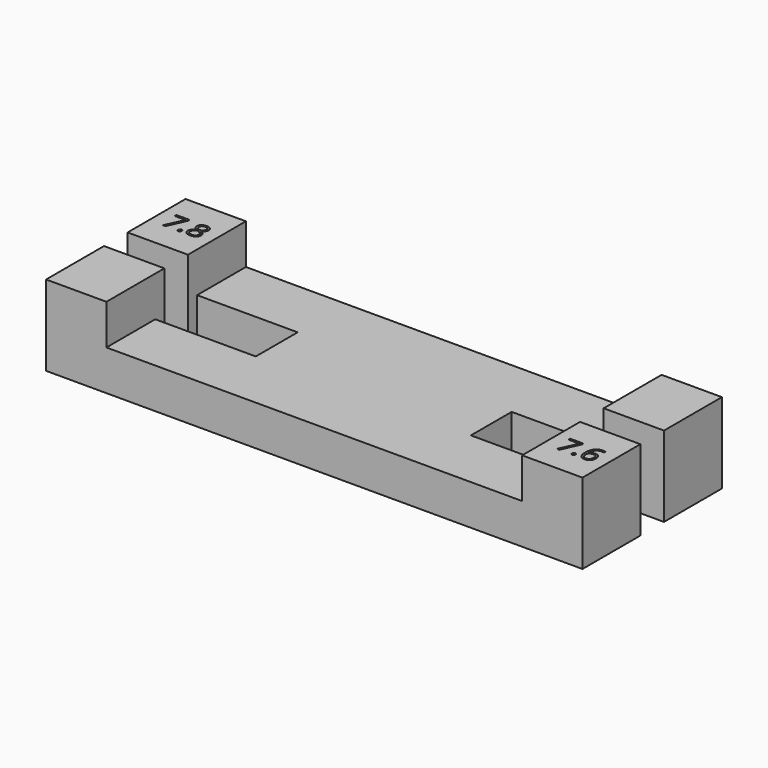
from build123d import *

# Parameters (mm, degrees)
F1_DEPTH     = 12
F2_W         = 62
F2_H         = 5
F3_DEPTH     = 6
F4_W         = 15
F4_H         = 1.7
F4_H_2       = 1.6
F5_DEPTH     = 25
F6_TEXT_SIZE = 4.1666666667
F7_DEPTH     = 5
F8_TEXT_SIZE = 4.1666666667
F9_DEPTH     = 5


# Not quite as in the source:
# - Text() gives the source's letters only with a copy of the font that has no kerning and outlines rounded to 1/6400 em; it was checked with that copy


with BuildPart() as f1:
    # F0 (on Top) → F1 (new body)
    with BuildSketch(Plane.XY):
        Polygon((40, 2.2), (40, 13), (-40, 13), (-40, 2.2), (-16, 2.2), (-16, -2.2), (-40, -2.2), (-40, -13), (40, -13), (40, -2.2), (16, -2.2), (16, 2.2), align=None)
    extrude(amount=F1_DEPTH)

    # F2 (on face) → F3 (cut)
    with BuildSketch(Plane.XY.offset(12)):
        with Locations((0, 10.5)):
            Rectangle(F2_W, F2_H)
        Polygon((31, 8), (-31, 8), (-31, 2.2), (-16, 2.2), (-16, -2.2), (-31, -2.2), (-31, -8), (31, -8), (31, -2.2), (16, -2.2), (16, 2.2), (31, 2.2), align=None)
        with Locations((0, -10.5)):
            Rectangle(F2_W, F2_H)
    extrude(amount=-F3_DEPTH, mode=Mode.SUBTRACT)

    # F4 (on face) → F5 (cut)
    with BuildSketch(Plane.XY.offset(6)):
        with Locations((-23.5, 3.05)):
            Rectangle(F4_W, F4_H)
        with Locations((-23.5, -3.05)):
            Rectangle(F4_W, F4_H)
        with Locations((23.5, 3)):
            Rectangle(F4_W, F4_H_2)
        with Locations((23.5, -3)):
            Rectangle(F4_W, F4_H_2)
    extrude(amount=-F5_DEPTH, mode=Mode.SUBTRACT)

    # F6 (on face) → F7 (cut)
    with BuildSketch(Plane.XY.offset(12)):
        with Locations((-38.5, 6.2)):
            Text('7.8', F6_TEXT_SIZE, font='Open Sans', text_align=(TextAlign.LEFT, TextAlign.BOTTOM))
    extrude(amount=-F7_DEPTH, mode=Mode.SUBTRACT)

    # F8 (on face) → F9 (cut)
    with BuildSketch(Plane.XY.offset(12)):
        with Locations((32.5598958333, -9.2)):
            Text('7.6', F8_TEXT_SIZE, font='Open Sans', text_align=(TextAlign.LEFT, TextAlign.BOTTOM))
    extrude(amount=-F9_DEPTH, mode=Mode.SUBTRACT)


solid = f1.part
